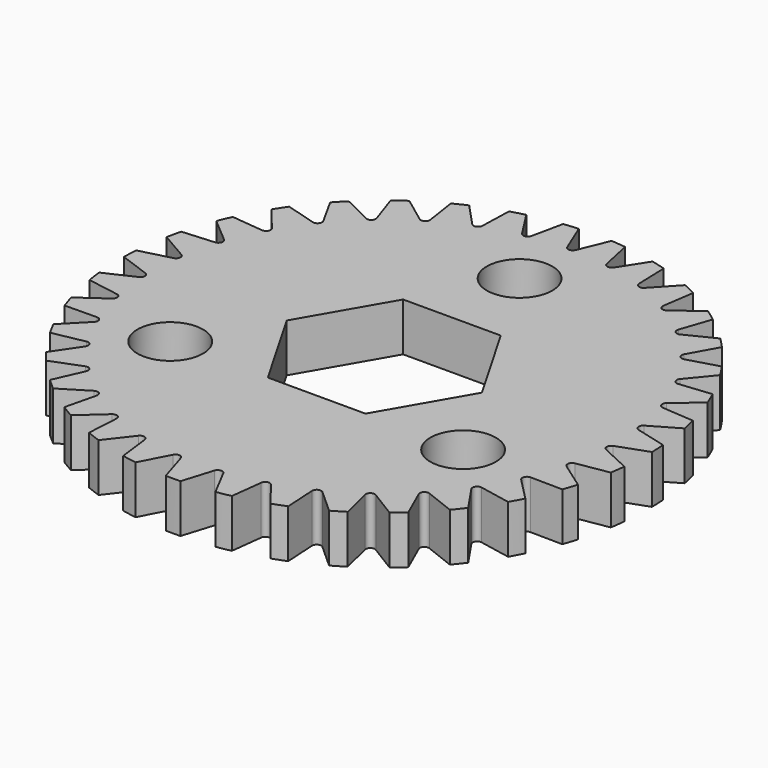
from build123d import *

# Parameters (mm, degrees)
F0_R            = 17.3565013667
F0_R_2          = 2.15265
F1_DEPTH        = 3.175
F3_DEPTH        = 3.175
F3_COPIES_COUNT = 35


# Not quite as in the source:
# - a pattern or mirror of a feature is missing from the dataset's text; its kind, count and spacing are read off the source's solid
# - a feature names something its author has since deleted; it is built from what else it names


with BuildPart() as f1:
    # F0 (on Top) → F1 (new body)
    with BuildSketch(Plane.XY):
        Circle(F0_R)
        with Locations((-9.6237072996, -5.55625)):
            Circle(F0_R_2, mode=Mode.SUBTRACT)
        with Locations((9.6237072996, -5.55625)):
            Circle(F0_R_2, mode=Mode.SUBTRACT)
        Polygon((6.4158048664, 0), (3.2079024332, -5.55625), (-3.2079024332, -5.55625), (-6.4158048664, 0), (-3.2079024332, 5.55625), (3.2079024332, 5.55625), align=None, mode=Mode.SUBTRACT)
        with Locations((0, 11.1125)):
            Circle(F0_R_2, mode=Mode.SUBTRACT)
    extrude(amount=F1_DEPTH)

    # F2 (on face) → F3 (cut, through all)
    with BuildSketch(Plane.XY.offset(3.175)):
        with BuildLine():
            Line((0.275157943, 15.3777549622), (1.0756124971, 17.3231405192))
            ThreePointArc((1.0756124971, 17.3231405192), (0, 17.3565013667), (-1.0756124971, 17.3231405192))
            Line((-1.0756124971, 17.3231405192), (-0.275157943, 15.3777549622))
            ThreePointArc((-0.275157943, 15.3777549622), (0, 15.1934323047), (0.275157943, 15.3777549622))
        make_face()
    f3 = extrude(amount=-F3_DEPTH, mode=Mode.SUBTRACT)

    # F3_copies: F3 ×35 about axis
    f3_copies_axis = Axis((0, 0, 0), (0, 0, 1))
    for i in range(1, F3_COPIES_COUNT):
        add(f3.rotate(f3_copies_axis, i * 360 / F3_COPIES_COUNT), mode=Mode.SUBTRACT)


solid = f1.part
